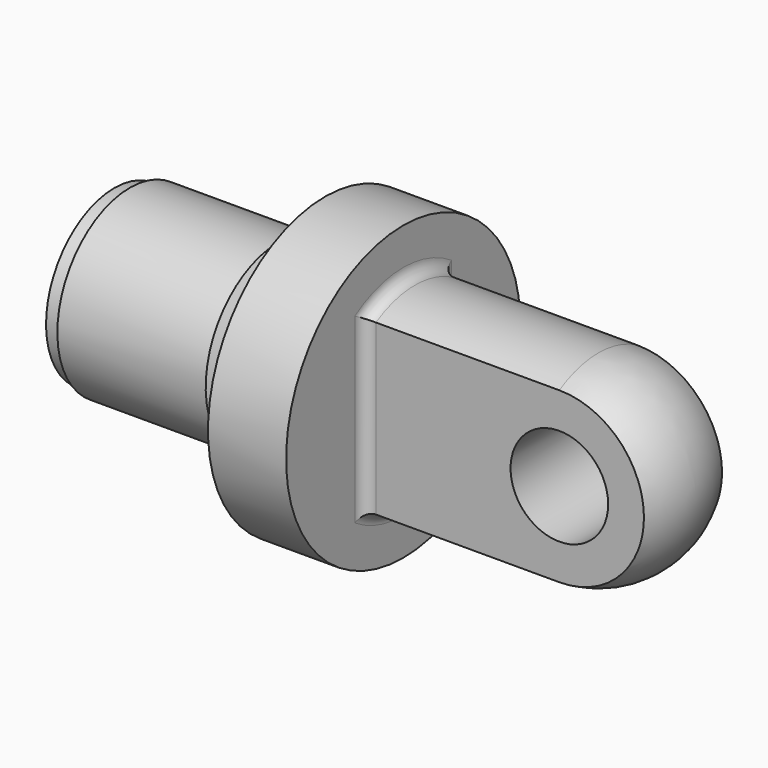
from build123d import *

# Parameters (mm, degrees)
F1_W     = 4
F1_H     = 21.875
F3_W     = 25
F3_H     = 43.3012701892
F4_DEPTH = 75
F5_R     = 12.5
F6_DEPTH = 25
F7_R     = 3


# Not quite as in the source:
# - a feature names something its author has since deleted; it is built from what else it names


with BuildPart() as f2:
    # F1 (on Front) → F2 (revolve)
    with BuildSketch(Plane.XZ):
        with BuildLine():
            Line((0, 21.875), (0, 0))
            Line((0, 0), (145, 0))
            ThreePointArc((145, 0), (137.6776695297, 17.6776695297), (120, 25))
            Line((120, 25), (70, 25))
            Line((70, 25), (70, 37.5))
            Line((70, 37.5), (50, 37.5))
            Line((50, 37.5), (50, 20.75))
            Line((50, 20.75), (39.443375673, 20.75))
            Line((39.443375673, 20.75), (38, 20.75))
            Line((38, 20.75), (38, 23.25))
            Line((38, 23.25), (0, 23.25))
            Line((0, 23.25), (0, 21.875))
        make_face()
        Polygon((39.443375673, 20.75), (38, 23.25), (38, 20.75), align=None)
        with Locations((-2, 10.9375)):
            Rectangle(F1_W, F1_H)
    revolve(axis=Axis((72.5, 0, 0), (-1, 0, 0)))

    # F3 (on face) → F4 (cut)
    with BuildSketch(Plane.YZ.offset(70)):
        with Locations((-25, 0)):
            Rectangle(F3_W, F3_H)
        with Locations((25, 0)):
            Rectangle(F3_W, F3_H)
    extrude(amount=F4_DEPTH, mode=Mode.SUBTRACT)

    # F5 (on face) → F6 (cut, through all)
    with BuildSketch(Plane.XZ.offset(12.5)):
        with Locations((120, 0)):
            Circle(F5_R)
    extrude(amount=-F6_DEPTH, mode=Mode.SUBTRACT)

    # F7
    f7_edges = [f2.edges().sort_by_distance(p)[0] for p in [
        (70, -12.5, 0),
        (70, 12.5, 0),
        (70, 0, 25),
        (70, 0, -25),
    ]]
    fillet(f7_edges, radius=F7_R)


solid = f2.part
